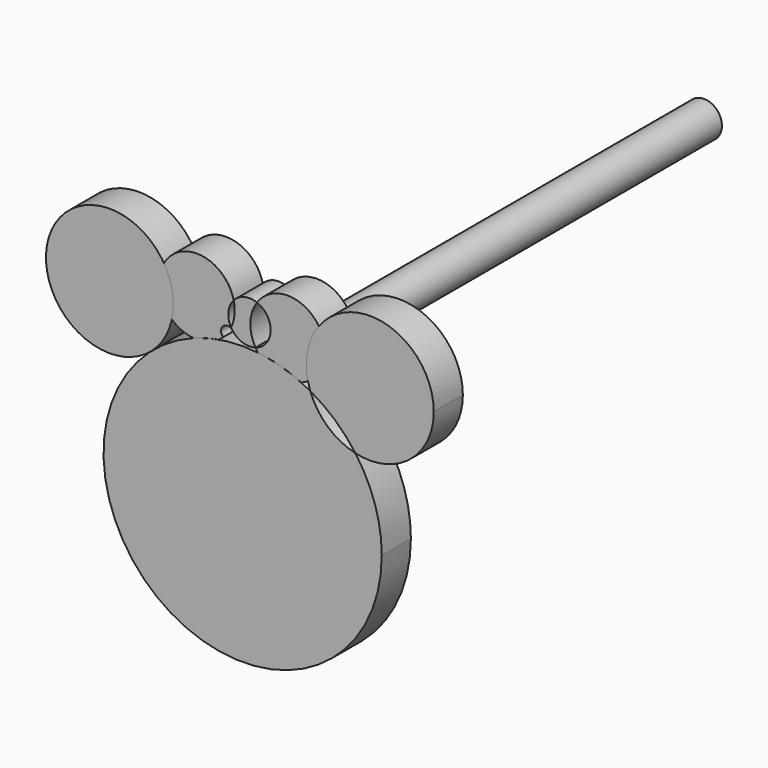
from build123d import *

# Parameters (mm, degrees)
F2_DEPTH = 25.4
F3_R     = 12.5347954463
F4_DEPTH = 368.2506931


# Not quite as in the source:
# - an extrude ends at something that could not be found from the text; its depth is read off the source's solid


with BuildPart() as f2:
    # F1 (on face) → F2 (new body)
    with BuildSketch(Plane.XZ):
        with BuildLine():
            ThreePointArc((8.9615103374, 93.3914722681), (5.3811386715, 107.5617064877), (9.9891173988, 121.4318590159))
            ThreePointArc((9.9891173988, 121.4318590159), (1.2641159909, 121.9639433995), (-6.2393266144, 117.4798479024))
            ThreePointArc((-6.2393266144, 117.4798479024), (-5.7205661899, 114.4957292899), (-5.5468846049, 111.4718392491))
            ThreePointArc((-5.5468846049, 111.4718392491), (-6.1846894375, 105.7027105797), (-8.0672985226, 100.2122257523))
            ThreePointArc((-8.0672985226, 100.2122257523), (-7.5718801063, 99.4100885879), (-7.0263945394, 98.6411224418))
            ThreePointArc((-7.0263945394, 98.6411224418), (0.1488565511, 93.5229275418), (8.9615103374, 93.3914722681))
        make_face()
    extrude(amount=-F2_DEPTH)


with BuildPart() as f2b:
    # F1 (on face) → F2, piece 2 (new body)
    with BuildSketch(Plane.XZ):
        with BuildLine():
            ThreePointArc((-8.0672985226, 100.2122257523), (-9.9517851493, 109.1422866074), (-6.2393266144, 117.4798479024))
            ThreePointArc((-6.2393266144, 117.4798479024), (-51.8998380867, 128.7872680092), (-34.2974279466, 85.1650808261))
            ThreePointArc((-34.2974279466, 85.1650808261), (-25.5546829871, 88.0009981982), (-16.5829647685, 89.9975674992))
            ThreePointArc((-16.5829647685, 89.9975674992), (-15.0203225596, 91.2072718845), (-13.5525071705, 92.5304322511))
            ThreePointArc((-13.5525071705, 92.5304322511), (-14.2405775832, 98.5709102582), (-8.2805496008, 99.7704442906))
            ThreePointArc((-8.2805496008, 99.7704442906), (-8.1728983191, 99.9908398881), (-8.0672985226, 100.2122257523))
        make_face()
    extrude(amount=-F2_DEPTH)


with BuildPart() as f2c:
    # F1 (on face) → F2, piece 3 (new body)
    with BuildSketch(Plane.XZ):
        with BuildLine():
            ThreePointArc((9.9891173988, 121.4318590159), (16.9384458795, 116.0025356672), (19.5658465826, 107.5842529502))
            ThreePointArc((19.5658465826, 107.5842529502), (16.6219789041, 98.7258251736), (8.9615103374, 93.3914722681))
            ThreePointArc((8.9615103374, 93.3914722681), (9.7806833027, 92.088163609), (10.6753514703, 90.8354758274))
            ThreePointArc((10.6753514703, 90.8354758274), (26.1768230416, 87.8290553094), (40.9860344784, 82.3498727218))
            ThreePointArc((40.9860344784, 82.3498727218), (52.9823213515, 91.9334549759), (57.5038948022, 106.6069453955))
            ThreePointArc((57.5038948022, 106.6069453955), (39.1986453542, 131.493850263), (9.9891173988, 121.4318590159))
        make_face()
    extrude(amount=-F2_DEPTH)


with BuildPart() as f2d:
    # F0 (on Front) → F2, piece 4 (new body)
    with BuildSketch(Plane.XZ):
        with BuildLine():
            ThreePointArc((-48.3549493189, 101.2052206791), (-133.2475901104, 119.6496048056), (-63.6618247207, 67.6421339817))
            ThreePointArc((-63.6618247207, 67.6421339817), (-52.3623085273, 82.7608365526), (-48.3549493189, 101.2052206791))
        make_face()
    extrude(amount=-F2_DEPTH)


with BuildPart() as f2e:
    # F0 (on Front) → F2, piece 5 (new body)
    with BuildSketch(Plane.XZ):
        with BuildLine():
            ThreePointArc((-63.6618247207, 67.6421339817), (-40.2909122509, -94.019991492), (97.0989918611, -5.674891965))
            ThreePointArc((97.0989918611, -5.674891965), (92.3900481259, 24.1963856734), (78.7199498001, 51.1703692615))
            ThreePointArc((78.7199498001, 51.1703692616), (59.4029165337, 61.2009472273), (47.1640406419, 79.2001190263))
            ThreePointArc((47.1640406419, 79.2001190263), (-10.071791025, 90.9003286974), (-63.6618247207, 67.6421339817))
        make_face()
    extrude(amount=-F2_DEPTH)

    # F3 (on face) → F4 (join, through all)
    with BuildSketch(Plane(origin=(0, 25.4, 0), x_dir=(-1, 0, 0), z_dir=(0, 1, 0))):
        with Locations((-7.0632169954, 73.0502381921)):
            Circle(F3_R)
    extrude(amount=F4_DEPTH)


with BuildPart() as f2f:
    # F0 (on Front) → F2, piece 6 (new body)
    with BuildSketch(Plane.XZ):
        with BuildLine():
            ThreePointArc((47.1640406419, 79.2001190263), (64.4834201975, 66.9205813104), (78.7199498001, 51.1703692615))
            ThreePointArc((78.7199498001, 51.1703692616), (116.5112316164, 59.5819602105), (133.3721522419, 94.4337205573))
            ThreePointArc((133.3721522419, 94.4337205573), (81.1873465112, 138.205575445), (47.1640406419, 79.2001190263))
        make_face()
    extrude(amount=-F2_DEPTH)


solid = Compound([f2.part, f2b.part, f2c.part, f2d.part, f2e.part, f2f.part])
